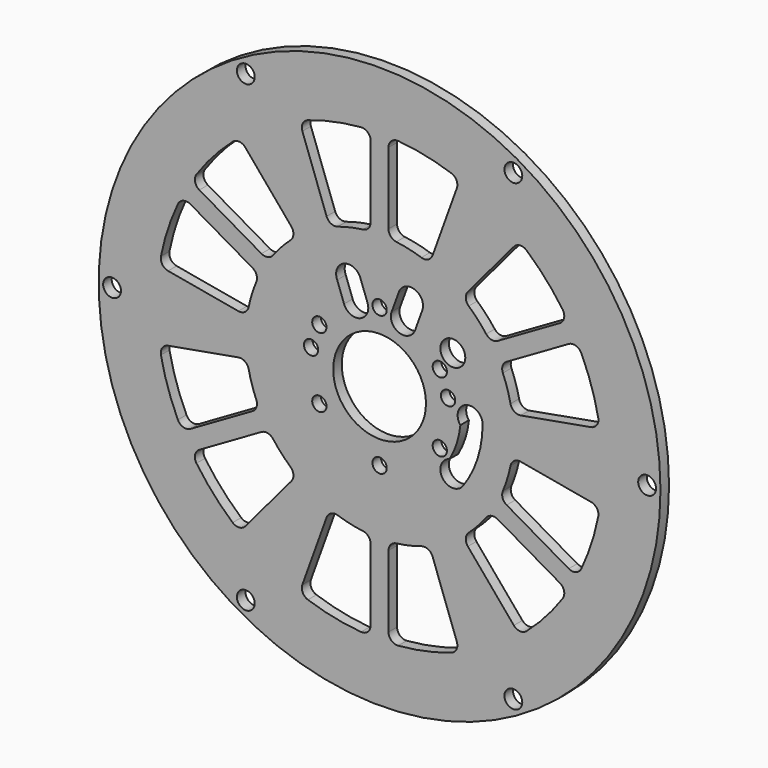
from build123d import *

# Parameters (mm, degrees)
F0_R     = 157.5
F0_R_2   = 5
F0_R_3   = 4
F0_R_4   = 26
F0_R_5   = 7
F1_DEPTH = 6


with BuildPart() as f1:
    # F0 (on Front) → F1 (new body)
    with BuildSketch(Plane.XZ):
        with Locations((-91.1300895214, 167.6714122295)):
            Circle(F0_R)
        with Locations((-166.1300895214, 37.7676016619)):
            Circle(F0_R_2, mode=Mode.SUBTRACT)
        with BuildLine():
            ThreePointArc((-120.8344120773, 93.3779815978), (-118.3207530584, 96.174141653), (-114.569425962, 96.4281844305))
            ThreePointArc((-114.569425962, 96.4281844305), (-107.6135679514, 94.5051977665), (-100.5050895214, 93.2596566058))
            ThreePointArc((-100.5050895214, 93.2596566058), (-97.3800895214, 91.6060620364), (-96.1300895214, 88.2988728976))
            Line((-96.1300895214, 88.2988728976), (-96.1300895214, 48.0888047985))
            ThreePointArc((-96.1300895214, 48.0888047985), (-97.7450735195, 44.4089044376), (-101.5467561881, 43.1061961556))
            ThreePointArc((-101.5467561881, 43.1061961556), (-116.6325114221, 45.3005559066), (-131.3389616262, 49.3149734353))
            ThreePointArc((-131.3389616262, 49.3149734353), (-134.2366143848, 51.8822295743), (-134.432970428, 55.7485766743))
            Line((-134.432970428, 55.7485766743), (-120.8344120773, 93.3779815978))
        make_face(mode=Mode.SUBTRACT)
        with BuildLine():
            ThreePointArc((-170.3222490608, 156.2493948493), (-166.6438739105, 155.4705823101), (-164.5482028633, 152.3488591354))
            ThreePointArc((-164.5482028633, 152.3488591354), (-162.7356291601, 145.3634160611), (-160.2600602317, 138.5845225782))
            ThreePointArc((-160.2600602317, 138.5845225782), (-160.1296151364, 135.0513959066), (-162.3687249457, 132.3152695825))
            Line((-162.3687249457, 132.3152695825), (-197.1916654074, 112.210235533))
            ThreePointArc((-197.1916654074, 112.210235533), (-201.1860446025, 111.7689025215), (-204.2150644027, 114.4099021486))
            ThreePointArc((-204.2150644027, 114.4099021486), (-209.8575707302, 128.5717292921), (-213.7342082711, 143.3150975327))
            ThreePointArc((-213.7342082711, 143.3150975327), (-212.959725616, 147.1081665025), (-209.7095488291, 149.2113893741))
            Line((-209.7095488291, 149.2113893741), (-170.3222490608, 156.2493948493))
        make_face(mode=Mode.SUBTRACT)
        with BuildLine():
            ThreePointArc((-157.3687249457, 123.6550155446), (-153.8796151364, 124.2260783593), (-150.8850602317, 122.3465462572))
            ThreePointArc((-150.8850602317, 122.3465462572), (-146.2521507301, 116.8131939349), (-141.1088664227, 111.7507375246))
            ThreePointArc((-141.1088664227, 111.7507375246), (-139.4532103734, 108.3749715724), (-140.6179265048, 104.799998978))
            Line((-140.6179265048, 104.799998978), (-166.4066679226, 74.2085995298))
            ThreePointArc((-166.4066679226, 74.2085995298), (-169.8532007526, 72.4454753013), (-173.5253361663, 73.6712881321))
            ThreePointArc((-173.5253361663, 73.6712881321), (-184.3551488295, 84.400238844), (-193.798397736, 96.3677062365))
            ThreePointArc((-193.798397736, 96.3677062365), (-194.5710606044, 100.3114141456), (-192.1916654074, 103.5499814951))
            Line((-192.1916654074, 103.5499814951), (-157.3687249457, 123.6550155446))
        make_face(mode=Mode.SUBTRACT)
        with Locations((-124.905080269, 148.1714122295)):
            Circle(F0_R_3, mode=Mode.SUBTRACT)
        with Locations((-16.1300895214, 37.7676016619)):
            Circle(F0_R_2, mode=Mode.SUBTRACT)
        with BuildLine():
            ThreePointArc((-67.6907530809, 96.4281844305), (-63.9394259844, 96.174141653), (-61.4257669655, 93.3779815978))
            Line((-61.4257669655, 93.3779815978), (-47.8272086148, 55.7485766743))
            ThreePointArc((-47.8272086148, 55.7485766743), (-48.023564658, 51.8822295743), (-50.9212174166, 49.3149734353))
            ThreePointArc((-50.9212174166, 49.3149734353), (-65.6276676207, 45.3005559066), (-80.7134228547, 43.1061961556))
            ThreePointArc((-80.7134228547, 43.1061961556), (-84.5151055233, 44.4089044376), (-86.1300895214, 48.0888047985))
            Line((-86.1300895214, 48.0888047985), (-86.1300895214, 88.2988728976))
            ThreePointArc((-86.1300895214, 88.2988728976), (-84.8800895214, 91.6060620364), (-81.7550895214, 93.2596566058))
            ThreePointArc((-81.7550895214, 93.2596566058), (-74.6466110914, 94.5051977665), (-67.6907530809, 96.4281844305))
        make_face(mode=Mode.SUBTRACT)
        with BuildLine():
            ThreePointArc((-41.642252538, 104.799998978), (-42.8069686694, 108.3749715724), (-41.1513126201, 111.7507375246))
            ThreePointArc((-41.1513126201, 111.7507375246), (-36.0080283127, 116.8131939349), (-31.3751188111, 122.3465462572))
            ThreePointArc((-31.3751188111, 122.3465462572), (-28.3805639064, 124.2260783593), (-24.8914540971, 123.6550155446))
            Line((-24.8914540971, 123.6550155446), (9.9314863646, 103.5499814951))
            ThreePointArc((9.9314863646, 103.5499814951), (12.3108815616, 100.3114141456), (11.5382186932, 96.3677062365))
            ThreePointArc((11.5382186932, 96.3677062365), (2.0949697867, 84.400238844), (-8.7348428765, 73.6712881321))
            ThreePointArc((-8.7348428765, 73.6712881321), (-12.4069782903, 72.4454753013), (-15.8535111203, 74.2085995298))
            Line((-15.8535111203, 74.2085995298), (-41.642252538, 104.799998978))
        make_face(mode=Mode.SUBTRACT)
        with Locations((-91.1300895214, 128.6714122295)):
            Circle(F0_R_3, mode=Mode.SUBTRACT)
        with Locations((-57.3550987738, 148.1714122295)):
            Circle(F0_R_3, mode=Mode.SUBTRACT)
        with BuildLine():
            ThreePointArc((-45.841296418, 163.2924603877), (-42.7008169638, 174.2755188412), (-33.3800895214, 167.6714122295))
            ThreePointArc((-33.3800895214, 167.6714122295), (-36.2065757054, 149.8256808044), (-44.4093580963, 133.7268139096))
            ThreePointArc((-44.4093580963, 133.7268139096), (-55.831781468, 133.8625655595), (-51.9168029329, 144.5939740068))
            ThreePointArc((-51.9168029329, 144.5939740068), (-47.85701803, 153.6111389855), (-45.841296418, 163.2924603877))
        make_face(mode=Mode.SUBTRACT)
        with BuildLine():
            ThreePointArc((-19.8914540971, 132.3152695825), (-22.1305639064, 135.0513959066), (-22.0001188111, 138.5845225782))
            ThreePointArc((-22.0001188111, 138.5845225782), (-19.5245498827, 145.3634160611), (-17.7119761796, 152.3488591354))
            ThreePointArc((-17.7119761796, 152.3488591354), (-15.6163051324, 155.4705823101), (-11.9379299821, 156.2493948493))
            Line((-11.9379299821, 156.2493948493), (27.4493697863, 149.2113893741))
            ThreePointArc((27.4493697863, 149.2113893741), (30.6995465732, 147.1081665025), (31.4740292283, 143.3150975327))
            ThreePointArc((31.4740292283, 143.3150975327), (27.5973916874, 128.5717292921), (21.9548853599, 114.4099021486))
            ThreePointArc((21.9548853599, 114.4099021486), (18.9258655597, 111.7689025215), (14.9314863646, 112.210235533))
            Line((14.9314863646, 112.210235533), (-19.8914540971, 132.3152695825))
        make_face(mode=Mode.SUBTRACT)
        with Locations((58.8699104786, 167.6714122295)):
            Circle(F0_R_2, mode=Mode.SUBTRACT)
        with Locations((-241.1300895214, 167.6714122295)):
            Circle(F0_R_2, mode=Mode.SUBTRACT)
        with BuildLine():
            ThreePointArc((-162.3687249457, 203.0275548766), (-160.1296151364, 200.2914285524), (-160.2600602317, 196.7583018809))
            ThreePointArc((-160.2600602317, 196.7583018809), (-162.7356291601, 189.9794083979), (-164.5482028633, 182.9939653237))
            ThreePointArc((-164.5482028633, 182.9939653237), (-166.6438739105, 179.872242149), (-170.3222490608, 179.0934296098))
            Line((-170.3222490608, 179.0934296098), (-209.7095488291, 186.131435085))
            ThreePointArc((-209.7095488291, 186.131435085), (-212.959725616, 188.2346579566), (-213.7342082711, 192.0277269264))
            ThreePointArc((-213.7342082711, 192.0277269264), (-209.8575707302, 206.7710951669), (-204.2150644027, 220.9329223104))
            ThreePointArc((-204.2150644027, 220.9329223104), (-201.1860446025, 223.5739219376), (-197.1916654074, 223.1325889261))
            Line((-197.1916654074, 223.1325889261), (-162.3687249457, 203.0275548766))
        make_face(mode=Mode.SUBTRACT)
        with Locations((-129.5375918889, 174.4436911585)):
            Circle(F0_R_3, mode=Mode.SUBTRACT)
        with Locations((-124.905080269, 187.1714122295)):
            Circle(F0_R_3, mode=Mode.SUBTRACT)
        with BuildLine():
            ThreePointArc((-140.6179265048, 230.542825481), (-139.4532103734, 226.9678528866), (-141.1088664227, 223.5920869344))
            ThreePointArc((-141.1088664227, 223.5920869344), (-146.2521507301, 218.5296305242), (-150.8850602317, 212.9962782019))
            ThreePointArc((-150.8850602317, 212.9962782019), (-153.8796151364, 211.1167460997), (-157.3687249457, 211.6878089144))
            Line((-157.3687249457, 211.6878089144), (-192.1916654074, 231.792842964))
            ThreePointArc((-192.1916654074, 231.792842964), (-194.5710606044, 235.0314103135), (-193.798397736, 238.9751182226))
            ThreePointArc((-193.798397736, 238.9751182226), (-184.3551488295, 250.942585615), (-173.5253361663, 261.6715363269))
            ThreePointArc((-173.5253361663, 261.6715363269), (-169.8532007526, 262.8973491577), (-166.4066679226, 261.1342249293))
            Line((-166.4066679226, 261.1342249293), (-140.6179265048, 230.542825481))
        make_face(mode=Mode.SUBTRACT)
        with BuildLine():
            ThreePointArc((-114.8846854021, 212.5187273615), (-110.8817527985, 221.9386610799), (-101.7603118429, 217.2956086804))
            Line((-101.7603118429, 217.2956086804), (-97.8945770466, 206.7232973485))
            ThreePointArc((-97.8945770466, 206.7232973485), (-102.0747340089, 197.7415761307), (-111.0502592598, 201.9350203873))
            Line((-111.0502592598, 201.9350203873), (-114.8846854021, 212.5187273615))
        make_face(mode=Mode.SUBTRACT)
        with BuildLine():
            ThreePointArc((-96.1300895214, 247.0439515615), (-97.3800895214, 243.7367624226), (-100.5050895214, 242.0831678532))
            ThreePointArc((-100.5050895214, 242.0831678532), (-107.6135679514, 240.8376266925), (-114.569425962, 238.9146400286))
            ThreePointArc((-114.569425962, 238.9146400286), (-118.3207530584, 239.1686828061), (-120.8344120773, 241.9648428613))
            Line((-120.8344120773, 241.9648428613), (-134.432970428, 279.5942477848))
            ThreePointArc((-134.432970428, 279.5942477848), (-134.2366143848, 283.4605948848), (-131.3389616262, 286.0278510238))
            ThreePointArc((-131.3389616262, 286.0278510238), (-116.6325114221, 290.0422685524), (-101.5467561881, 292.2366283035))
            ThreePointArc((-101.5467561881, 292.2366283035), (-97.7450735195, 290.9339200215), (-96.1300895214, 287.2540196606))
            Line((-96.1300895214, 287.2540196606), (-96.1300895214, 247.0439515615))
        make_face(mode=Mode.SUBTRACT)
        with Locations((-166.1300895214, 297.5752227972)):
            Circle(F0_R_2, mode=Mode.SUBTRACT)
        with Locations((-91.1300895214, 167.6714122295)):
            Circle(F0_R_4, mode=Mode.SUBTRACT)
        with Locations((-52.7225871539, 174.4436911585)):
            Circle(F0_R_3, mode=Mode.SUBTRACT)
        with Locations((-57.3550987738, 187.1714122295)):
            Circle(F0_R_3, mode=Mode.SUBTRACT)
        with Locations((-91.1300895214, 206.6714122295)):
            Circle(F0_R_3, mode=Mode.SUBTRACT)
        with Locations((-50.0724770569, 197.5015137834)):
            Circle(F0_R_5, mode=Mode.SUBTRACT)
        with BuildLine():
            Line((-84.3656019962, 206.7232973485), (-80.4998671999, 217.2956086804))
            ThreePointArc((-80.4998671999, 217.2956086804), (-71.3784262444, 221.9386610799), (-67.3754936407, 212.5187273615))
            Line((-67.3754936407, 212.5187273615), (-71.2099195621, 201.935020997))
            ThreePointArc((-71.2099195621, 201.935020997), (-80.1854447293, 197.7415760198), (-84.3656019962, 206.7232973485))
        make_face(mode=Mode.SUBTRACT)
        with BuildLine():
            ThreePointArc((-24.8914540971, 211.6878089144), (-28.3805639064, 211.1167460997), (-31.3751188111, 212.9962782019))
            ThreePointArc((-31.3751188111, 212.9962782019), (-36.0080283127, 218.5296305242), (-41.1513126201, 223.5920869344))
            ThreePointArc((-41.1513126201, 223.5920869344), (-42.8069686694, 226.9678528866), (-41.642252538, 230.542825481))
            Line((-41.642252538, 230.542825481), (-15.8535111203, 261.1342249293))
            ThreePointArc((-15.8535111203, 261.1342249293), (-12.4069782903, 262.8973491577), (-8.7348428765, 261.6715363269))
            ThreePointArc((-8.7348428765, 261.6715363269), (2.0949697867, 250.942585615), (11.5382186932, 238.9751182226))
            ThreePointArc((11.5382186932, 238.9751182226), (12.3108815616, 235.0314103135), (9.9314863646, 231.792842964))
            Line((9.9314863646, 231.792842964), (-24.8914540971, 211.6878089144))
        make_face(mode=Mode.SUBTRACT)
        with BuildLine():
            ThreePointArc((-11.9379299821, 179.0934296098), (-15.6163051324, 179.872242149), (-17.7119761796, 182.9939653237))
            ThreePointArc((-17.7119761796, 182.9939653237), (-19.5245498827, 189.9794083979), (-22.0001188111, 196.7583018809))
            ThreePointArc((-22.0001188111, 196.7583018809), (-22.1305639064, 200.2914285524), (-19.8914540971, 203.0275548766))
            Line((-19.8914540971, 203.0275548766), (14.9314863646, 223.1325889261))
            ThreePointArc((14.9314863646, 223.1325889261), (18.9258655597, 223.5739219376), (21.9548853599, 220.9329223104))
            ThreePointArc((21.9548853599, 220.9329223104), (27.5973916874, 206.7710951669), (31.4740292283, 192.0277269264))
            ThreePointArc((31.4740292283, 192.0277269264), (30.6995465732, 188.2346579566), (27.4493697863, 186.131435085))
            Line((27.4493697863, 186.131435085), (-11.9379299821, 179.0934296098))
        make_face(mode=Mode.SUBTRACT)
        with BuildLine():
            ThreePointArc((-61.4257669655, 241.9648428613), (-63.9394259844, 239.1686828061), (-67.6907530809, 238.9146400286))
            ThreePointArc((-67.6907530809, 238.9146400286), (-74.6466110914, 240.8376266925), (-81.7550895214, 242.0831678532))
            ThreePointArc((-81.7550895214, 242.0831678532), (-84.8800895214, 243.7367624226), (-86.1300895214, 247.0439515615))
            Line((-86.1300895214, 247.0439515615), (-86.1300895214, 287.2540196606))
            ThreePointArc((-86.1300895214, 287.2540196606), (-84.5151055233, 290.9339200215), (-80.7134228547, 292.2366283035))
            ThreePointArc((-80.7134228547, 292.2366283035), (-65.6276676207, 290.0422685524), (-50.9212174166, 286.0278510238))
            ThreePointArc((-50.9212174166, 286.0278510238), (-48.023564658, 283.4605948848), (-47.8272086148, 279.5942477848))
            Line((-47.8272086148, 279.5942477848), (-61.4257669655, 241.9648428613))
        make_face(mode=Mode.SUBTRACT)
        with Locations((-16.1300895214, 297.5752227972)):
            Circle(F0_R_2, mode=Mode.SUBTRACT)
    extrude(amount=F1_DEPTH)


solid = f1.part
